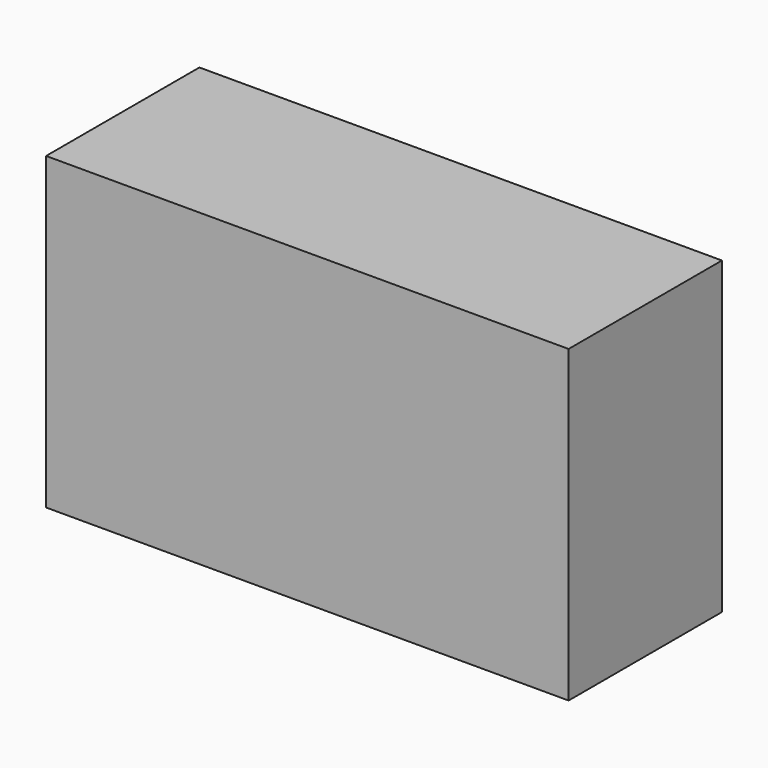
from build123d import *

# Parameters (mm, degrees)
F0_W     = 83.8060937822
F0_H     = 49.6412403882
F1_DEPTH = 30.734


# Not quite as in the source:
# - the program builds the solid bodies; features that only make, move or delete a surface that nothing else refers to are left out


with BuildPart() as f1:
    # F0 (on Front) → F1 (new body)
    with BuildSketch(Plane.XZ):
        with Locations((3.7960950285, 10.0742522627)):
            Rectangle(F0_W, F0_H)
    extrude(amount=F1_DEPTH)


solid = f1.part
